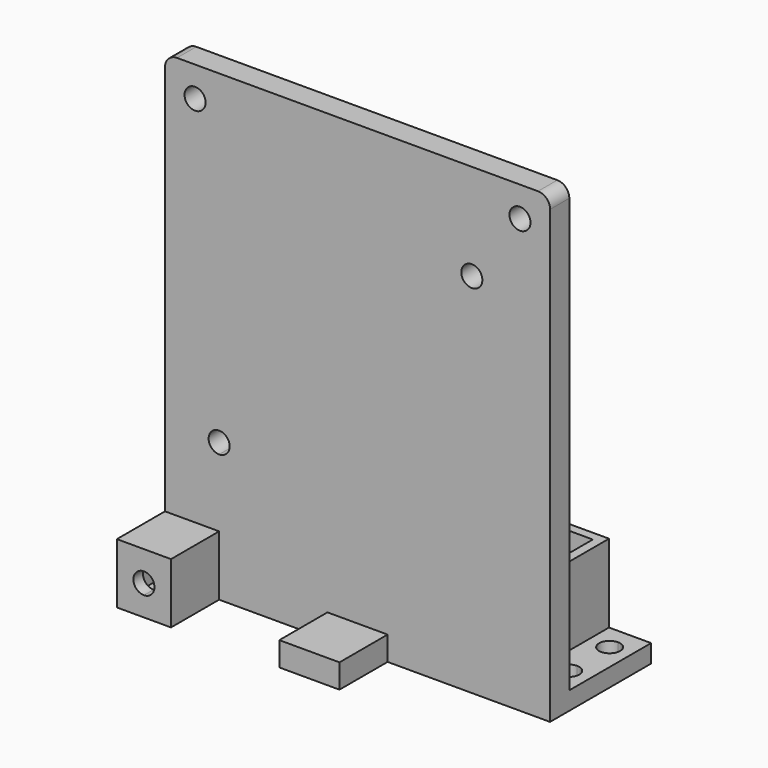
from build123d import *

# Parameters (mm, degrees)
F0_W      = 64
F0_H      = 77
F1_DEPTH  = 4
F2_R      = 1.75
F3_DEPTH  = 25
F5_DEPTH  = 10
F7_DEPTH  = 25
F8_W      = 21.5
F8_H      = 16
F9_DEPTH  = 17
F10_W     = 18.5
F10_H     = 15.5
F11_DEPTH = 25
F12_W     = 17
F12_H     = 3
F13_DEPTH = 7
F14_W     = 17
F14_H     = 3
F15_DEPTH = 7
F17_DEPTH = 25
F19_DEPTH = 25
F21_DEPTH = 10
F22_DEPTH = 25
F23_W     = 5.5
F23_H     = 6
F23_R     = 1.75
F24_DEPTH = 12
F25_R     = 2


# Not quite as in the source:
# - a feature names something its author has since deleted; it is built from what else it names


with BuildPart() as f1:
    # F0 (on Front) → F1 (new body)
    with BuildSketch(Plane.XZ):
        Rectangle(F0_W, F0_H)
    extrude(amount=F1_DEPTH)

    # F2 (on face) → F3 (cut)
    with BuildSketch(Plane.XZ.offset(4)):
        with BuildLine():
            ThreePointArc((-28.75, 33.5), (-27, 31.75), (-25.25, 33.5))
            ThreePointArc((-25.25, 33.5), (-27, 35.25), (-28.75, 33.5))
        make_face()
        with Locations((27, 33.5)):
            Circle(F2_R)
    extrude(amount=-F3_DEPTH, mode=Mode.SUBTRACT)

    # F4 (on face) → F5 (join)
    with BuildSketch(Plane.XZ.offset(4)):
        Polygon((-5, -34.5), (-5, -38.5), (0, -38.5), (5, -38.5), (5, -34.5), align=None)
    extrude(amount=F5_DEPTH)

    # F6 (on face) → F7 (cut)
    with BuildSketch(Plane.XZ.offset(4)):
        with BuildLine():
            Line((19, 22.5), (19, 24.25))
            ThreePointArc((19, 24.25), (17.7625631329, 21.2625631329), (20.75, 22.5))
            Line((20.75, 22.5), (19, 22.5))
        make_face()
        with BuildLine():
            ThreePointArc((20.75, 22.5), (20.2374368671, 23.7374368671), (19, 24.25))
            Line((19, 24.25), (19, 22.5))
            Line((19, 22.5), (20.75, 22.5))
        make_face()
        with BuildLine():
            ThreePointArc((-21.25, -15.5), (-24.2374368671, -14.2625631329), (-23, -17.25))
            ThreePointArc((-23, -17.25), (-21.7625631329, -16.7374368671), (-21.25, -15.5))
        make_face()
    extrude(amount=-F7_DEPTH, mode=Mode.SUBTRACT)

    # F8 (on face) → F9 (join)
    with BuildSketch(Plane(origin=(0, 0, 0), x_dir=(-1, 0, 0), z_dir=(0, 1, 0))):
        with Locations((-14.25, -30.5)):
            Rectangle(F8_W, F8_H)
    extrude(amount=F9_DEPTH)

    # F10 (on face) → F11 (cut)
    with BuildSketch(Plane.XY.offset(-22.5)):
        with Locations((14.25, 7.75)):
            Rectangle(F10_W, F10_H)
    extrude(amount=-F11_DEPTH, mode=Mode.SUBTRACT)

    # F12 (on face) → F13 (join)
    with BuildSketch(Plane.YZ.offset(25)):
        with Locations((8.5, -37)):
            Rectangle(F12_W, F12_H)
    extrude(amount=F13_DEPTH)

    # F14 (on face) → F15 (join)
    with BuildSketch(Plane(origin=(3.5, 0, 0), x_dir=(0, -1, 0), z_dir=(-1, 0, 0))):
        with Locations((-8.5, -37)):
            Rectangle(F14_W, F14_H)
    extrude(amount=F15_DEPTH)

    # F16 (on face) → F17 (cut)
    with BuildSketch(Plane.XY.offset(-35.5)):
        with BuildLine():
            Line((0, 14.5), (0, 11))
            ThreePointArc((0, 11), (1.2374368671, 11.5125631329), (1.75, 12.75))
            ThreePointArc((1.75, 12.75), (1.2374368671, 13.9874368671), (0, 14.5))
        make_face()
        with BuildLine():
            ThreePointArc((0, 14.5), (-1.75, 12.75), (0, 11))
            Line((0, 11), (0, 14.5))
        make_face()
        with BuildLine():
            ThreePointArc((0, 6), (-1.75, 4.25), (0, 2.5))
            Line((0, 2.5), (0, 6))
        make_face()
        with BuildLine():
            Line((0, 6), (0, 2.5))
            ThreePointArc((0, 2.5), (1.2374368671, 3.0125631329), (1.75, 4.25))
            ThreePointArc((1.75, 4.25), (1.2374368671, 5.4874368671), (0, 6))
        make_face()
    extrude(amount=-F17_DEPTH, mode=Mode.SUBTRACT)

    # F18 (on face) → F19 (cut)
    with BuildSketch(Plane.XY.offset(-35.5)):
        with BuildLine():
            ThreePointArc((30.25, 12.75), (29.7374368671, 13.9874368671), (28.5, 14.5))
            Line((28.5, 14.5), (28.5, 11))
            ThreePointArc((28.5, 11), (29.7374368671, 11.5125631329), (30.25, 12.75))
        make_face()
        with BuildLine():
            ThreePointArc((30.25, 4.25), (29.7374368671, 5.4874368671), (28.5, 6))
            Line((28.5, 6), (28.5, 2.5))
            ThreePointArc((28.5, 2.5), (29.7374368671, 3.0125631329), (30.25, 4.25))
        make_face()
        with BuildLine():
            Line((28.5, 2.5), (28.5, 6))
            ThreePointArc((28.5, 6), (26.75, 4.25), (28.5, 2.5))
        make_face()
        with BuildLine():
            Line((28.5, 11), (28.5, 14.5))
            ThreePointArc((28.5, 14.5), (26.75, 12.75), (28.5, 11))
        make_face()
    extrude(amount=-F19_DEPTH, mode=Mode.SUBTRACT)

    # F20 (on face) → F21 (join)
    with BuildSketch(Plane.XZ.offset(4)):
        Polygon((-32, -28.5), (-32, -38.5), (-27.5, -38.5), (-23, -38.5), (-23, -28.5), align=None)
        with BuildLine():
            ThreePointArc((-25.75, -33.5), (-26.2625631329, -34.7374368671), (-27.5, -35.25))
            ThreePointArc((-27.5, -35.25), (-28.7374368671, -32.2625631329), (-25.75, -33.5))
        make_face(mode=Mode.SUBTRACT)
    extrude(amount=F21_DEPTH)

    # F22 (cut): a face of the model
    f22_faces = [f1.faces().sort_by_distance(p)[0] for p in [
        (-27.5, -4, -33.5),
    ]]
    extrude(f22_faces, amount=-F22_DEPTH, mode=Mode.SUBTRACT)

    # F23 (on face) → F24 (cut)
    with BuildSketch(Plane(origin=(0, 0, 0), x_dir=(-1, 0, 0), z_dir=(0, 1, 0))):
        with Locations((27.5, -33.5)):
            Rectangle(F23_W, F23_H)
        with Locations((27.5, -33.5)):
            Circle(F23_R, mode=Mode.SUBTRACT)
    extrude(amount=-F24_DEPTH, mode=Mode.SUBTRACT)

    # F25
    f25_edges = [f1.edges().sort_by_distance(p)[0] for p in [
        (-32, -2, 38.5),
        (32, -2, 38.5),
    ]]
    fillet(f25_edges, radius=F25_R)


solid = f1.part
